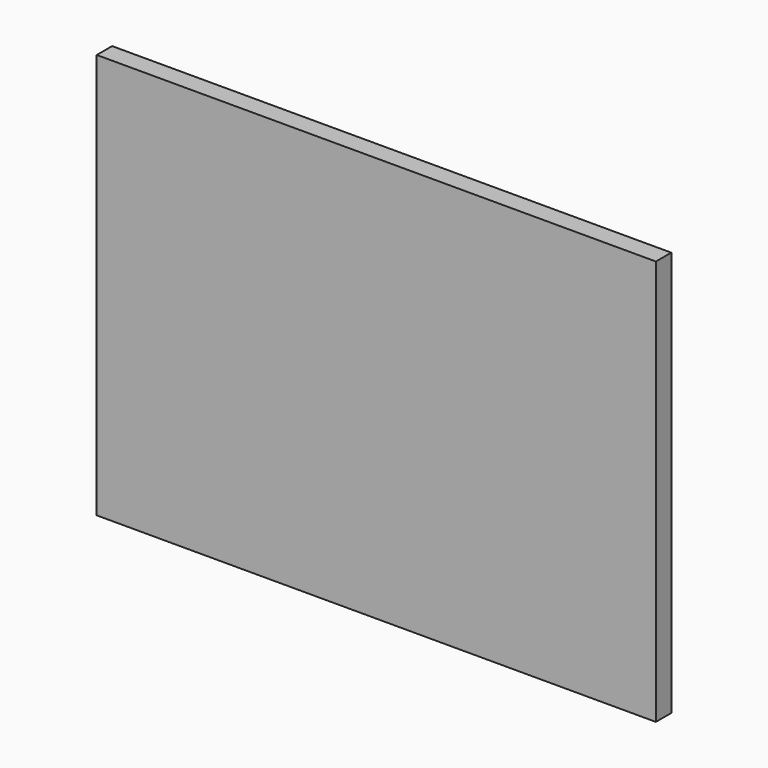
from build123d import *

# Parameters (mm, degrees)
F0_W        = 170.942
F0_H        = 120.142
F1_DEPTH    = 12.7
F2_W        = 184.658
F2_H        = 133.858
F2_W_2      = 170.942
F2_H_2      = 120.142
F3_DEPTH    = 6.35
F4_T        = 3.81
F4_T3_DEPTH = 127.762
F4_T5_DEPTH = 178.562


# Not quite as in the source:
# - a shell that OpenCascade refuses in one call is made with other operations: the cavity is built on its own and cut out


with BuildPart() as f1:
    # F0 (on Front) → F1 (new body)
    with BuildSketch(Plane.XZ):
        with Locations((85.471, 60.071)):
            Rectangle(F0_W, F0_H)
    extrude(amount=F1_DEPTH)

    # F2 (on face) → F3 (join)
    with BuildSketch(Plane.XZ.offset(12.7)):
        with Locations((85.471, 60.071)):
            Rectangle(F2_W, F2_H)
        with Locations((85.471, 60.071)):
            Rectangle(F2_W_2, F2_H_2, mode=Mode.SUBTRACT)
    extrude(amount=-F3_DEPTH)

    # F4: shell of thickness 3.81, made by hand


with BuildPart() as f4_core1:
    # F4_t2: copy of F1
    add(f1.part)

    # the walls: a layer under each face that stays
    f4_faces = [f4_core1.faces().sort_by_distance(p)[0] for p in [
        (0, -3.175, 60.071),
        (85.471, -3.175, 0),
        (-0.7027333333, -6.35, -2.3960666667),
        (85.471, -3.175, 120.142),
        (170.942, -3.175, 60.071),
        (-6.858, -9.525, 60.071),
        (85.471, -9.525, -6.858),
        (177.8, -9.525, 60.071),
        (85.471, -9.525, 127),
        (85.471, -12.7, 60.071),
    ]]
    thicken(f4_faces, amount=-F4_T, mode=Mode.SUBTRACT)

    # F4_s4 → F4_t3 (cut)
    with BuildSketch(Plane.XY.offset(-3.81)):
        Polygon((-0.0381, -6.3119), (3.81, -6.35), (3.81, -10.16), (0, -10.16), align=None)
        Polygon((170.9801, -6.3119), (170.942, -10.16), (167.132, -10.16), (167.132, -6.35), align=None)
    extrude(amount=F4_T3_DEPTH, mode=Mode.SUBTRACT)

    # F4_s6 → F4_t5 (cut)
    with BuildSketch(Plane.YZ.offset(-3.81)):
        Polygon((-6.3119, -0.0381), (-6.35, 3.81), (-10.16, 3.81), (-10.16, 0), align=None)
        Polygon((-6.3119, 120.1801), (-10.16, 120.142), (-10.16, 116.332), (-6.35, 116.332), align=None)
    extrude(amount=F4_T5_DEPTH, mode=Mode.SUBTRACT)


with BuildPart() as f1_1:
    add(f1.part)

    # what is left inside the walls is the cavity
    f4_cavity = [f4_core1.part.solids().sort_by_distance(p)[0] for p in [
        (85.471, -8.8519, 41.317333),
    ]]
    add(f4_cavity, mode=Mode.SUBTRACT)


solid = f1_1.part
